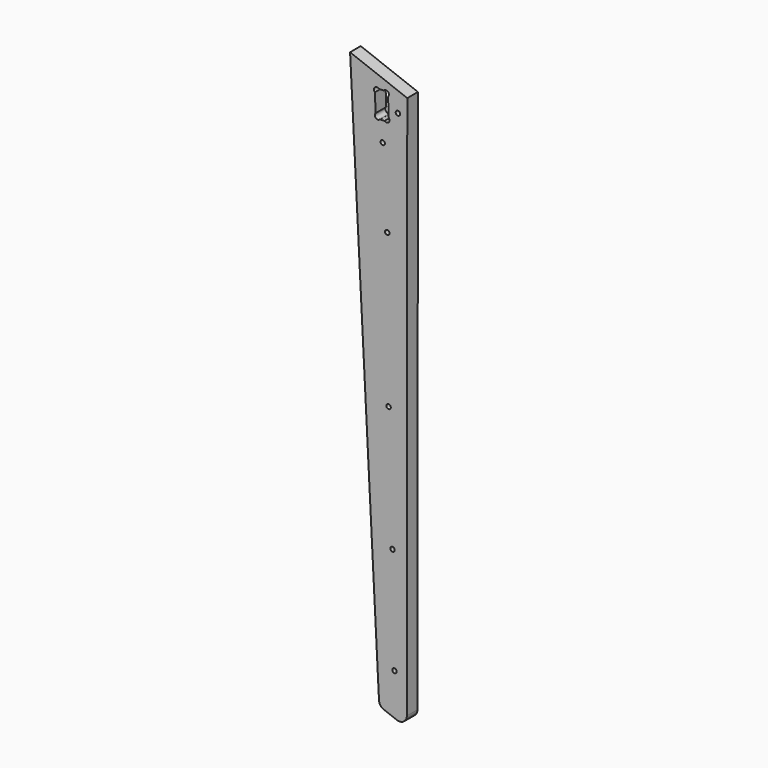
from build123d import *

# Parameters (mm, degrees)
F0_R     = 3
F1_DEPTH = 18
F2_DEPTH = 14


# Not quite as in the source:
# - ends of sketch curves that miss each other by under 0.0002 mm in the source are joined


with BuildPart() as f1:
    # F0 (on Front) → F1 (new body)
    with BuildSketch(Plane.XZ):
        with BuildLine():
            Line((-42.3895305789, -243.8882939158), (-24.7354158314, -250.6203213983))
            ThreePointArc((-24.7354158314, -250.6203213983), (-15.5028330705, -249.5140993631), (-11.1723924415, -241.2853938543))
            Line((-11.1723924415, -241.2853938543), (-10.5257942379, 495.2740080398))
            Line((-10.5257942379, 495.2740080398), (-87.9671722006, 524.8046568947))
            Line((-87.9671722006, 524.8046568947), (-48.8132548023, -235.0591811233))
            ThreePointArc((-48.8132548023, -235.0591811233), (-46.9127527413, -240.4278329279), (-42.3895305789, -243.8882939158))
        make_face()
        with Locations((-27.881012126, -192.8539189117)):
            Circle(F0_R, mode=Mode.SUBTRACT)
        with Locations((-30.5399937075, -49.059701124)):
            Circle(F0_R, mode=Mode.SUBTRACT)
        with Locations((-35.8245981399, 119.2769033151)):
            Circle(F0_R, mode=Mode.SUBTRACT)
        with Locations((-37.6148353963, 326.2889456799)):
            Circle(F0_R, mode=Mode.SUBTRACT)
        with BuildLine():
            ThreePointArc((-35.8713849562, 463.9863896495), (-35.6237850386, 458.3139596858), (-41.2978981422, 458.1085140717))
            Line((-41.2978981422, 458.1085140717), (-47.5773687005, 457.9045057833))
            ThreePointArc((-47.5773687005, 457.9045057833), (-53.2508540354, 457.7393262229), (-53.3777836629, 463.4137960782))
            Line((-53.3777836629, 463.4137960782), (-54.3935717097, 487.9983330149))
            ThreePointArc((-54.3935717097, 487.9983330149), (-54.636241933, 493.6693642066), (-48.9636796908, 493.8731318846))
            Line((-48.9636796908, 493.8731318846), (-42.2828997396, 494.0973559272))
            ThreePointArc((-42.2828997396, 494.0973559272), (-36.6071005964, 494.2603360531), (-36.4869165759, 488.5834695431))
            Line((-36.4869165759, 488.5834695431), (-35.8713849562, 463.9863896495))
        make_face(mode=Mode.SUBTRACT)
        with Locations((-43.7681841537, 431.407725542)):
            Circle(F0_R, mode=Mode.SUBTRACT)
        with Locations((-23.2091454593, 473.1308742023)):
            Circle(F0_R, mode=Mode.SUBTRACT)
        with Locations((-43.7681841537, 431.407725542)):
            Circle(F0_R)
        with Locations((-23.2091454593, 473.1308742023)):
            Circle(F0_R)
        with Locations((-37.6148353963, 326.2889456799)):
            Circle(F0_R)
        with Locations((-35.8245981399, 119.2769033151)):
            Circle(F0_R)
        with Locations((-27.881012126, -192.8539189117)):
            Circle(F0_R)
        with Locations((-30.5399937075, -49.059701124)):
            Circle(F0_R)
    extrude(amount=-F1_DEPTH)

    # F0 (on Front) → F2 (cut)
    with BuildSketch(Plane.XZ):
        with Locations((-43.7681841537, 431.407725542)):
            Circle(F0_R)
        with Locations((-23.2091454593, 473.1308742023)):
            Circle(F0_R)
        with Locations((-37.6148353963, 326.2889456799)):
            Circle(F0_R)
        with Locations((-35.8245981399, 119.2769033151)):
            Circle(F0_R)
        with Locations((-27.881012126, -192.8539189117)):
            Circle(F0_R)
        with Locations((-30.5399937075, -49.059701124)):
            Circle(F0_R)
    extrude(amount=-F2_DEPTH, mode=Mode.SUBTRACT)


solid = f1.part
